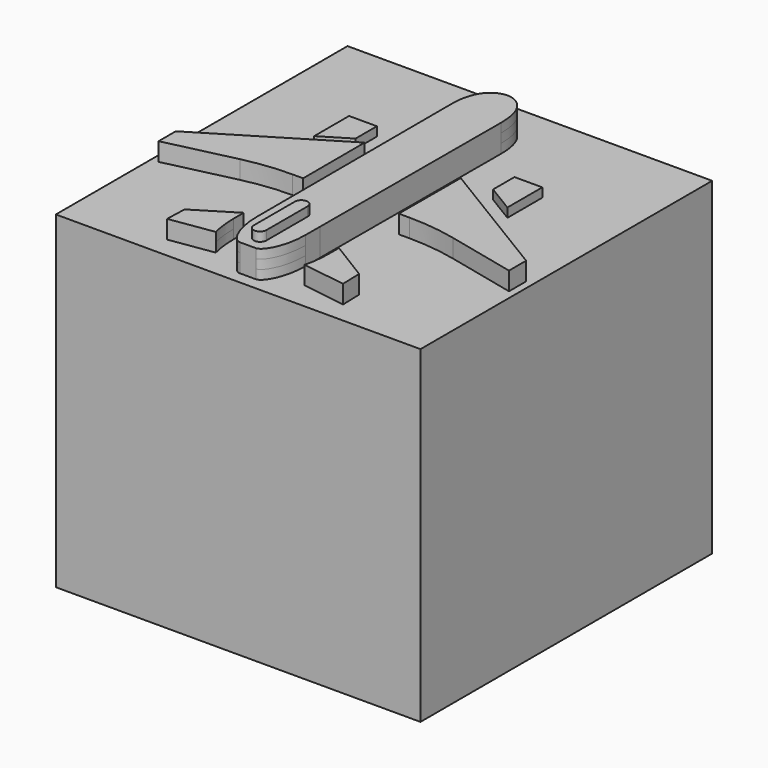
from build123d import *

# Parameters (mm, degrees)
F0_W     = 200
F0_H     = 200
F1_DEPTH = 180
F2_DEPTH = 185
F3_DEPTH = 190
F4_DEPTH = 195
F6_DEPTH = 5


# Not quite as in the source:
# - the dataset's text gives a spline's control points without its knots; the knots are read off the source's solid


with BuildPart() as f1:
    # F0 (on Top) → F1 (new body)
    with BuildSketch(Plane.XY):
        Rectangle(F0_W, F0_H)
        with BuildLine():
            Line((-47.8931178828, -76.908331888), (-26.1435569325, -63.5429788096))
            Line((-26.1435569325, -63.5429788096), (-26.1262354313, -70.5461896311))
            add(Edge.make_bspline(
                [(-26.1262354313, -70.5461896311), (-26.1301214344, -72.6447513101), (-25.9226885629, -76.7122275938), (-25.206617008, -81.3929883408), (-24.6039868813, -84.0128411258), (-24.3904465876, -84.8459593127)],
                knots=[0, 0, 0, 0, 0.125, 0.25, 0.31021936, 0.31021936, 0.31021936, 0.31021936], degree=3))
            Line((-24.3904465876, -84.8459593127), (-48.2336984492, -88.4332945935))
            Line((-48.2336984492, -88.4332945935), (-47.8931178828, -76.908331888))
        make_face(mode=Mode.SUBTRACT)
        with BuildLine():
            Line((-96.1022423344, -22.6553896196), (-26.3494160677, 19.6873894598))
            Line((-26.3494160677, 19.6873894598), (-26.2446868917, -22.6553896196))
            Line((-26.2446868917, -22.6553896196), (-31.9787403088, -22.6553896196))
            ThreePointArc((-31.9787403088, -22.6553896196), (-45.2780803321, -23.4148901061), (-58.4044897199, -25.6835158197))
            Line((-58.4044897199, -25.6835158197), (-96.0743982111, -34.4315737997))
            Line((-96.0743982111, -34.4315737997), (-96.1022423344, -22.6553896196))
        make_face(mode=Mode.SUBTRACT)
        with BuildLine():
            Line((26.1262354313, -70.5461896311), (26.1435569325, -63.5429788096))
            Line((26.1435569325, -63.5429788096), (47.8931178828, -76.908331888))
            Line((47.8931178828, -76.908331888), (48.2336984492, -88.4332945935))
            Line((48.2336984492, -88.4332945935), (24.3904465876, -84.8459593127))
            add(Edge.make_bspline(
                [(26.1262354313, -70.5461896311), (26.1301214344, -72.6447513101), (25.9226885629, -76.7122275938), (25.206617008, -81.3929883408), (24.6039868813, -84.0128411258), (24.3904465876, -84.8459593127)],
                knots=[0, 0, 0, 0, 0.125, 0.25, 0.31021936, 0.31021936, 0.31021936, 0.31021936], degree=3))
        make_face(mode=Mode.SUBTRACT)
        with BuildLine():
            Line((-13.4509153585, -60.5521906389), (-13.7433838099, 63.1422176957))
            add(Edge.make_bspline(
                [(0, 84.6024081111), (-2.034754958, 84.6024081111), (-13.7433838099, 83.4568068385), (-13.7433838099, 63.1422176957)],
                knots=[0, 0, 0, 0, 25.4837275769, 25.4837275769, 25.4837275769, 25.4837275769], degree=3))
            add(Edge.make_bspline(
                [(0, 84.6024081111), (2.034754958, 84.6024081111), (13.7433838099, 83.4568068385), (13.7433838099, 63.1422176957)],
                knots=[0, 0, 0, 0, 25.4837275769, 25.4837275769, 25.4837275769, 25.4837275769], degree=3))
            Line((13.7433838099, 63.1422176957), (13.4509153585, -60.5521906389))
            Line((13.4509153585, -60.5521906389), (13.4262572051, -70.569688655))
            add(Edge.make_bspline(
                [(13.4262572051, -70.569688655), (13.4509153585, -83.8858529803), (8.007301067, -93.3943380051), (4.3828436889, -93.3943312552)],
                knots=[0, 0, 0, 0, 24.5509192873, 24.5509192873, 24.5509192873, 24.5509192873], degree=3))
            Line((4.3828436889, -93.3943312552), (0, -93.3943312552))
            Line((0, -93.3943312552), (-4.3828436889, -93.3943312552))
            add(Edge.make_bspline(
                [(-13.4262572051, -70.569688655), (-13.4509153585, -83.8858529803), (-8.007301067, -93.3943380051), (-4.3828436889, -93.3943312552)],
                knots=[0, 0, 0, 0, 24.5509192873, 24.5509192873, 24.5509192873, 24.5509192873], degree=3))
            Line((-13.4262572051, -70.569688655), (-13.4509153585, -60.5521906389))
        make_face(mode=Mode.SUBTRACT)
        with BuildLine():
            Line((26.2446868917, -22.6553896196), (26.3494160677, 19.6873894598))
            Line((26.3494160677, 19.6873894598), (96.1022423344, -22.6553896196))
            Line((96.1022423344, -22.6553896196), (96.0743982111, -34.4315737997))
            Line((96.0743982111, -34.4315737997), (58.4044897199, -25.6835158197))
            ThreePointArc((58.4044897199, -25.6835158197), (45.2780803321, -23.4148901061), (31.9787403088, -22.6553896196))
            Line((31.9787403088, -22.6553896196), (26.2446868917, -22.6553896196))
        make_face(mode=Mode.SUBTRACT)
        Polygon((-52.9935426026, 42.2937646508), (-37.7366803586, 42.2937646508), (-37.7366803586, 27.6316785991), (-52.9935426026, 18.3701478193), align=None, mode=Mode.SUBTRACT)
        Polygon((52.9935426026, 18.3701478193), (37.7366803586, 27.6316785991), (37.7366803586, 42.2937646508), (52.9935426026, 42.2937646508), align=None, mode=Mode.SUBTRACT)
        Polygon((-37.7366803586, 27.6316785991), (-37.7366803586, 42.2937646508), (-52.9935426026, 42.2937646508), (-52.9935426026, 18.3701478193), align=None)
        with BuildLine():
            add(Edge.make_bspline(
                [(0, 84.6024081111), (-2.034754958, 84.6024081111), (-13.7433838099, 83.4568068385), (-13.7433838099, 63.1422176957)],
                knots=[0, 0, 0, 0, 25.4837275769, 25.4837275769, 25.4837275769, 25.4837275769], degree=3))
            Line((-13.7433838099, 63.1422176957), (-13.4509153585, -60.5521906389))
            Line((-13.4509153585, -60.5521906389), (-13.4262572051, -70.569688655))
            add(Edge.make_bspline(
                [(-13.4262572051, -70.569688655), (-13.4509153585, -83.8858529803), (-8.007301067, -93.3943380051), (-4.3828436889, -93.3943312552)],
                knots=[0, 0, 0, 0, 24.5509192873, 24.5509192873, 24.5509192873, 24.5509192873], degree=3))
            Line((-4.3828436889, -93.3943312552), (0, -93.3943312552))
            Line((0, -93.3943312552), (4.3828436889, -93.3943312552))
            add(Edge.make_bspline(
                [(13.4262572051, -70.569688655), (13.4509153585, -83.8858529803), (8.007301067, -93.3943380051), (4.3828436889, -93.3943312552)],
                knots=[0, 0, 0, 0, 24.5509192873, 24.5509192873, 24.5509192873, 24.5509192873], degree=3))
            Line((13.4262572051, -70.569688655), (13.4509153585, -60.5521906389))
            Line((13.4509153585, -60.5521906389), (13.7433838099, 63.1422176957))
            add(Edge.make_bspline(
                [(0, 84.6024081111), (2.034754958, 84.6024081111), (13.7433838099, 83.4568068385), (13.7433838099, 63.1422176957)],
                knots=[0, 0, 0, 0, 25.4837275769, 25.4837275769, 25.4837275769, 25.4837275769], degree=3))
        make_face()
        with BuildLine():
            Line((-26.2446868917, -22.6553896196), (-26.3494160677, 19.6873894598))
            Line((-26.3494160677, 19.6873894598), (-96.1022423344, -22.6553896196))
            Line((-96.1022423344, -22.6553896196), (-96.0743982111, -34.4315737997))
            Line((-96.0743982111, -34.4315737997), (-58.4044897199, -25.6835158197))
            ThreePointArc((-58.4044897199, -25.6835158197), (-45.2780803321, -23.4148901061), (-31.9787403088, -22.6553896196))
            Line((-31.9787403088, -22.6553896196), (-26.2446868917, -22.6553896196))
        make_face()
        with BuildLine():
            Line((96.1022423344, -22.6553896196), (26.3494160677, 19.6873894598))
            Line((26.3494160677, 19.6873894598), (26.2446868917, -22.6553896196))
            Line((26.2446868917, -22.6553896196), (31.9787403088, -22.6553896196))
            ThreePointArc((31.9787403088, -22.6553896196), (45.2780803321, -23.4148901061), (58.4044897199, -25.6835158197))
            Line((58.4044897199, -25.6835158197), (96.0743982111, -34.4315737997))
            Line((96.0743982111, -34.4315737997), (96.1022423344, -22.6553896196))
        make_face()
        Polygon((37.7366803586, 42.2937646508), (37.7366803586, 27.6316785991), (52.9935426026, 18.3701478193), (52.9935426026, 42.2937646508), align=None)
        with BuildLine():
            Line((47.8931178828, -76.908331888), (26.1435569325, -63.5429788096))
            Line((26.1435569325, -63.5429788096), (26.1262354313, -70.5461896311))
            add(Edge.make_bspline(
                [(26.1262354313, -70.5461896311), (26.1301214344, -72.6447513101), (25.9226885629, -76.7122275938), (25.206617008, -81.3929883408), (24.6039868813, -84.0128411258), (24.3904465876, -84.8459593127)],
                knots=[0, 0, 0, 0, 0.125, 0.25, 0.31021936, 0.31021936, 0.31021936, 0.31021936], degree=3))
            Line((24.3904465876, -84.8459593127), (48.2336984492, -88.4332945935))
            Line((48.2336984492, -88.4332945935), (47.8931178828, -76.908331888))
        make_face()
        with BuildLine():
            Line((-26.1262354313, -70.5461896311), (-26.1435569325, -63.5429788096))
            Line((-26.1435569325, -63.5429788096), (-47.8931178828, -76.908331888))
            Line((-47.8931178828, -76.908331888), (-48.2336984492, -88.4332945935))
            Line((-48.2336984492, -88.4332945935), (-24.3904465876, -84.8459593127))
            add(Edge.make_bspline(
                [(-26.1262354313, -70.5461896311), (-26.1301214344, -72.6447513101), (-25.9226885629, -76.7122275938), (-25.206617008, -81.3929883408), (-24.6039868813, -84.0128411258), (-24.3904465876, -84.8459593127)],
                knots=[0, 0, 0, 0, 0.125, 0.25, 0.31021936, 0.31021936, 0.31021936, 0.31021936], degree=3))
        make_face()
    extrude(amount=F1_DEPTH)

    # F0 (on Top) → F2 (join)
    with BuildSketch(Plane.XY):
        with BuildLine():
            add(Edge.make_bspline(
                [(0, 84.6024081111), (-2.034754958, 84.6024081111), (-13.7433838099, 83.4568068385), (-13.7433838099, 63.1422176957)],
                knots=[0, 0, 0, 0, 25.4837275769, 25.4837275769, 25.4837275769, 25.4837275769], degree=3))
            Line((-13.7433838099, 63.1422176957), (-13.4509153585, -60.5521906389))
            Line((-13.4509153585, -60.5521906389), (-13.4262572051, -70.569688655))
            add(Edge.make_bspline(
                [(-13.4262572051, -70.569688655), (-13.4509153585, -83.8858529803), (-8.007301067, -93.3943380051), (-4.3828436889, -93.3943312552)],
                knots=[0, 0, 0, 0, 24.5509192873, 24.5509192873, 24.5509192873, 24.5509192873], degree=3))
            Line((-4.3828436889, -93.3943312552), (0, -93.3943312552))
            Line((0, -93.3943312552), (4.3828436889, -93.3943312552))
            add(Edge.make_bspline(
                [(13.4262572051, -70.569688655), (13.4509153585, -83.8858529803), (8.007301067, -93.3943380051), (4.3828436889, -93.3943312552)],
                knots=[0, 0, 0, 0, 24.5509192873, 24.5509192873, 24.5509192873, 24.5509192873], degree=3))
            Line((13.4262572051, -70.569688655), (13.4509153585, -60.5521906389))
            Line((13.4509153585, -60.5521906389), (13.7433838099, 63.1422176957))
            add(Edge.make_bspline(
                [(0, 84.6024081111), (2.034754958, 84.6024081111), (13.7433838099, 83.4568068385), (13.7433838099, 63.1422176957)],
                knots=[0, 0, 0, 0, 25.4837275769, 25.4837275769, 25.4837275769, 25.4837275769], degree=3))
        make_face()
        with BuildLine():
            Line((-26.2446868917, -22.6553896196), (-26.3494160677, 19.6873894598))
            Line((-26.3494160677, 19.6873894598), (-96.1022423344, -22.6553896196))
            Line((-96.1022423344, -22.6553896196), (-96.0743982111, -34.4315737997))
            Line((-96.0743982111, -34.4315737997), (-58.4044897199, -25.6835158197))
            ThreePointArc((-58.4044897199, -25.6835158197), (-45.2780803321, -23.4148901061), (-31.9787403088, -22.6553896196))
            Line((-31.9787403088, -22.6553896196), (-26.2446868917, -22.6553896196))
        make_face()
        with BuildLine():
            Line((-26.1262354313, -70.5461896311), (-26.1435569325, -63.5429788096))
            Line((-26.1435569325, -63.5429788096), (-47.8931178828, -76.908331888))
            Line((-47.8931178828, -76.908331888), (-48.2336984492, -88.4332945935))
            Line((-48.2336984492, -88.4332945935), (-24.3904465876, -84.8459593127))
            add(Edge.make_bspline(
                [(-26.1262354313, -70.5461896311), (-26.1301214344, -72.6447513101), (-25.9226885629, -76.7122275938), (-25.206617008, -81.3929883408), (-24.6039868813, -84.0128411258), (-24.3904465876, -84.8459593127)],
                knots=[0, 0, 0, 0, 0.125, 0.25, 0.31021936, 0.31021936, 0.31021936, 0.31021936], degree=3))
        make_face()
        with BuildLine():
            Line((47.8931178828, -76.908331888), (26.1435569325, -63.5429788096))
            Line((26.1435569325, -63.5429788096), (26.1262354313, -70.5461896311))
            add(Edge.make_bspline(
                [(26.1262354313, -70.5461896311), (26.1301214344, -72.6447513101), (25.9226885629, -76.7122275938), (25.206617008, -81.3929883408), (24.6039868813, -84.0128411258), (24.3904465876, -84.8459593127)],
                knots=[0, 0, 0, 0, 0.125, 0.25, 0.31021936, 0.31021936, 0.31021936, 0.31021936], degree=3))
            Line((24.3904465876, -84.8459593127), (48.2336984492, -88.4332945935))
            Line((48.2336984492, -88.4332945935), (47.8931178828, -76.908331888))
        make_face()
        with BuildLine():
            Line((96.1022423344, -22.6553896196), (26.3494160677, 19.6873894598))
            Line((26.3494160677, 19.6873894598), (26.2446868917, -22.6553896196))
            Line((26.2446868917, -22.6553896196), (31.9787403088, -22.6553896196))
            ThreePointArc((31.9787403088, -22.6553896196), (45.2780803321, -23.4148901061), (58.4044897199, -25.6835158197))
            Line((58.4044897199, -25.6835158197), (96.0743982111, -34.4315737997))
            Line((96.0743982111, -34.4315737997), (96.1022423344, -22.6553896196))
        make_face()
        Polygon((37.7366803586, 42.2937646508), (37.7366803586, 27.6316785991), (52.9935426026, 18.3701478193), (52.9935426026, 42.2937646508), align=None)
        Polygon((-37.7366803586, 27.6316785991), (-37.7366803586, 42.2937646508), (-52.9935426026, 42.2937646508), (-52.9935426026, 18.3701478193), align=None)
    extrude(amount=F2_DEPTH)

    # F0 (on Top) → F3 (join)
    with BuildSketch(Plane.XY):
        with BuildLine():
            add(Edge.make_bspline(
                [(0, 84.6024081111), (-2.034754958, 84.6024081111), (-13.7433838099, 83.4568068385), (-13.7433838099, 63.1422176957)],
                knots=[0, 0, 0, 0, 25.4837275769, 25.4837275769, 25.4837275769, 25.4837275769], degree=3))
            Line((-13.7433838099, 63.1422176957), (-13.4509153585, -60.5521906389))
            Line((-13.4509153585, -60.5521906389), (-13.4262572051, -70.569688655))
            add(Edge.make_bspline(
                [(-13.4262572051, -70.569688655), (-13.4509153585, -83.8858529803), (-8.007301067, -93.3943380051), (-4.3828436889, -93.3943312552)],
                knots=[0, 0, 0, 0, 24.5509192873, 24.5509192873, 24.5509192873, 24.5509192873], degree=3))
            Line((-4.3828436889, -93.3943312552), (0, -93.3943312552))
            Line((0, -93.3943312552), (4.3828436889, -93.3943312552))
            add(Edge.make_bspline(
                [(13.4262572051, -70.569688655), (13.4509153585, -83.8858529803), (8.007301067, -93.3943380051), (4.3828436889, -93.3943312552)],
                knots=[0, 0, 0, 0, 24.5509192873, 24.5509192873, 24.5509192873, 24.5509192873], degree=3))
            Line((13.4262572051, -70.569688655), (13.4509153585, -60.5521906389))
            Line((13.4509153585, -60.5521906389), (13.7433838099, 63.1422176957))
            add(Edge.make_bspline(
                [(0, 84.6024081111), (2.034754958, 84.6024081111), (13.7433838099, 83.4568068385), (13.7433838099, 63.1422176957)],
                knots=[0, 0, 0, 0, 25.4837275769, 25.4837275769, 25.4837275769, 25.4837275769], degree=3))
        make_face()
        with BuildLine():
            Line((-26.2446868917, -22.6553896196), (-26.3494160677, 19.6873894598))
            Line((-26.3494160677, 19.6873894598), (-96.1022423344, -22.6553896196))
            Line((-96.1022423344, -22.6553896196), (-96.0743982111, -34.4315737997))
            Line((-96.0743982111, -34.4315737997), (-58.4044897199, -25.6835158197))
            ThreePointArc((-58.4044897199, -25.6835158197), (-45.2780803321, -23.4148901061), (-31.9787403088, -22.6553896196))
            Line((-31.9787403088, -22.6553896196), (-26.2446868917, -22.6553896196))
        make_face()
        with BuildLine():
            Line((-26.1262354313, -70.5461896311), (-26.1435569325, -63.5429788096))
            Line((-26.1435569325, -63.5429788096), (-47.8931178828, -76.908331888))
            Line((-47.8931178828, -76.908331888), (-48.2336984492, -88.4332945935))
            Line((-48.2336984492, -88.4332945935), (-24.3904465876, -84.8459593127))
            add(Edge.make_bspline(
                [(-26.1262354313, -70.5461896311), (-26.1301214344, -72.6447513101), (-25.9226885629, -76.7122275938), (-25.206617008, -81.3929883408), (-24.6039868813, -84.0128411258), (-24.3904465876, -84.8459593127)],
                knots=[0, 0, 0, 0, 0.125, 0.25, 0.31021936, 0.31021936, 0.31021936, 0.31021936], degree=3))
        make_face()
        with BuildLine():
            Line((47.8931178828, -76.908331888), (26.1435569325, -63.5429788096))
            Line((26.1435569325, -63.5429788096), (26.1262354313, -70.5461896311))
            add(Edge.make_bspline(
                [(26.1262354313, -70.5461896311), (26.1301214344, -72.6447513101), (25.9226885629, -76.7122275938), (25.206617008, -81.3929883408), (24.6039868813, -84.0128411258), (24.3904465876, -84.8459593127)],
                knots=[0, 0, 0, 0, 0.125, 0.25, 0.31021936, 0.31021936, 0.31021936, 0.31021936], degree=3))
            Line((24.3904465876, -84.8459593127), (48.2336984492, -88.4332945935))
            Line((48.2336984492, -88.4332945935), (47.8931178828, -76.908331888))
        make_face()
        with BuildLine():
            Line((96.1022423344, -22.6553896196), (26.3494160677, 19.6873894598))
            Line((26.3494160677, 19.6873894598), (26.2446868917, -22.6553896196))
            Line((26.2446868917, -22.6553896196), (31.9787403088, -22.6553896196))
            ThreePointArc((31.9787403088, -22.6553896196), (45.2780803321, -23.4148901061), (58.4044897199, -25.6835158197))
            Line((58.4044897199, -25.6835158197), (96.0743982111, -34.4315737997))
            Line((96.0743982111, -34.4315737997), (96.1022423344, -22.6553896196))
        make_face()
    extrude(amount=F3_DEPTH)

    # F0 (on Top) → F4 (join)
    with BuildSketch(Plane.XY):
        with BuildLine():
            add(Edge.make_bspline(
                [(0, 84.6024081111), (-2.034754958, 84.6024081111), (-13.7433838099, 83.4568068385), (-13.7433838099, 63.1422176957)],
                knots=[0, 0, 0, 0, 25.4837275769, 25.4837275769, 25.4837275769, 25.4837275769], degree=3))
            Line((-13.7433838099, 63.1422176957), (-13.4509153585, -60.5521906389))
            Line((-13.4509153585, -60.5521906389), (-13.4262572051, -70.569688655))
            add(Edge.make_bspline(
                [(-13.4262572051, -70.569688655), (-13.4509153585, -83.8858529803), (-8.007301067, -93.3943380051), (-4.3828436889, -93.3943312552)],
                knots=[0, 0, 0, 0, 24.5509192873, 24.5509192873, 24.5509192873, 24.5509192873], degree=3))
            Line((-4.3828436889, -93.3943312552), (0, -93.3943312552))
            Line((0, -93.3943312552), (4.3828436889, -93.3943312552))
            add(Edge.make_bspline(
                [(13.4262572051, -70.569688655), (13.4509153585, -83.8858529803), (8.007301067, -93.3943380051), (4.3828436889, -93.3943312552)],
                knots=[0, 0, 0, 0, 24.5509192873, 24.5509192873, 24.5509192873, 24.5509192873], degree=3))
            Line((13.4262572051, -70.569688655), (13.4509153585, -60.5521906389))
            Line((13.4509153585, -60.5521906389), (13.7433838099, 63.1422176957))
            add(Edge.make_bspline(
                [(0, 84.6024081111), (2.034754958, 84.6024081111), (13.7433838099, 83.4568068385), (13.7433838099, 63.1422176957)],
                knots=[0, 0, 0, 0, 25.4837275769, 25.4837275769, 25.4837275769, 25.4837275769], degree=3))
        make_face()
    extrude(amount=F4_DEPTH)

    # F5 (on face) → F6 (join)
    with BuildSketch(Plane.XY.offset(195)):
        with BuildLine():
            Line((3.494290635, -84.9771350622), (3.494290635, -56.7144453526))
            ThreePointArc((3.494290635, -56.7144453526), (0, -53.2201547176), (-3.494290635, -56.7144453526))
            Line((-3.494290635, -56.7144453526), (-3.494290635, -84.9771350622))
            ThreePointArc((-3.494290635, -84.9771350622), (0, -88.4714256972), (3.494290635, -84.9771350622))
        make_face()
    extrude(amount=F6_DEPTH)


solid = f1.part
